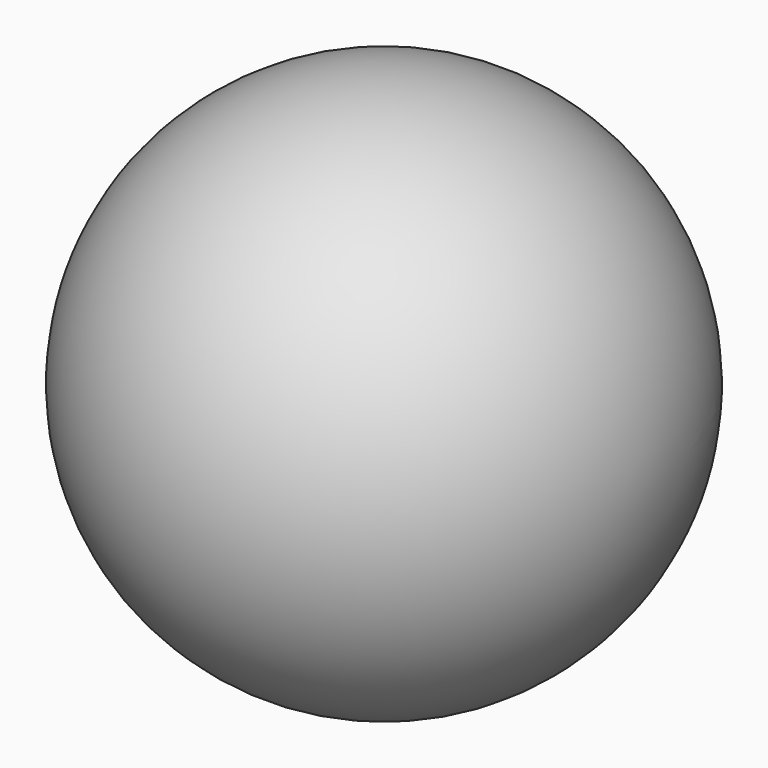
from build123d import *


with BuildPart() as f1:
    # F0 (on Top) → F1 (revolve)
    with BuildSketch(Plane.XY):
        with BuildLine():
            Line((0, 0), (5.9314720365, 0))
            ThreePointArc((5.9314720365, 0), (0, 5.9314720365), (-5.9314720365, 0))
            Line((-5.9314720365, 0), (0, 0))
        make_face()
    revolve(axis=Axis((0, 0, 0), (-1, 0, 0)))


solid = f1.part
